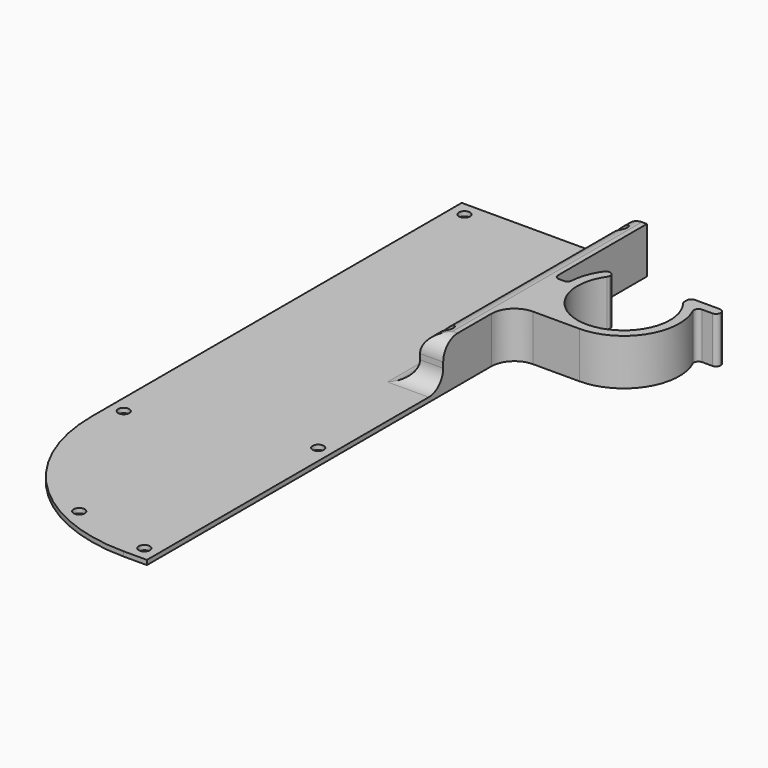
from build123d import *

# Parameters (mm, degrees)
F1_DEPTH     = 10
F3_DEPTH     = 9
F5_D         = 2.4
F6_T1_DEPTH  = 55
F6_T3_DEPTH  = 5
F6_T9_DEPTH  = 64.75
F6_T13_DEPTH = 14.75
F6_T16_DEPTH = 24.5
F6_T18_DEPTH = 74.5


# Not quite as in the source:
# - a fillet or chamfer that OpenCascade refuses, or shapes differently, is made with other operations: its cross-section is extruded or revolved along the edge and cut away or added
# - a feature names something its author has since deleted; it is built from what else it names


with BuildPart() as f1:
    # F0 (on Top) → F1 (new body)
    with BuildSketch(Plane.XY):
        with BuildLine():
            Line((-30, 0), (-70, 0))
            Line((-70, 0), (-70, -100))
            ThreePointArc((-70, -100), (-59.7487373415, -124.7487373415), (-35, -135))
            Line((-35, -135), (-30, -135))
            Line((-30, -135), (-30, -42))
            ThreePointArc((-30, -42), (-28.5355339059, -38.4644660941), (-25, -37))
            Line((-25, -37), (-15, -37))
            ThreePointArc((-15, -37), (-4.9050660078, -31.4878584828), (-4.0842494776, -20.0153846154))
            ThreePointArc((-4.0842494776, -20.0153846154), (-4.0158481001, -19.0593451264), (-3.1746036007, -18.6))
            Line((-3.1746036007, -18.6), (-1, -18.6))
            ThreePointArc((-1, -18.6), (-0.2928932188, -18.3071067812), (0, -17.6))
            ThreePointArc((0, -17.6), (-0.2928932188, -16.8928932188), (-1, -16.6))
            Line((-1, -16.6), (-6.3162509151, -16.6))
            ThreePointArc((-6.3162509151, -16.6), (-7.0233576963, -16.8928932188), (-7.3162509151, -17.6))
            Line((-7.3162509151, -17.6), (-7.3162509151, -18.2477780079))
            ThreePointArc((-7.3162509151, -18.2477780079), (-7.2621451309, -18.5722531726), (-7.1056826501, -18.8616163708))
            ThreePointArc((-7.1056826501, -18.8616163708), (-14.7582290616, -34.9970769134), (-23.1818181818, -19.2504042542))
            ThreePointArc((-23.1818181818, -19.2504042542), (-23.0465374108, -18.9769560242), (-23, -18.6754446797))
            ThreePointArc((-23, -18.6754446797), (-23.6984886554, -17.7219820904), (-24.8181818182, -18.1004851051))
            ThreePointArc((-24.8181818182, -18.1004851051), (-26.2938104102, -20.9441589751), (-26.9644443663, -24.0769230769))
            ThreePointArc((-26.9644443663, -24.0769230769), (-27.2821151763, -24.7337993857), (-27.9614813968, -25))
            Line((-27.9614813968, -25), (-29, -25))
            ThreePointArc((-29, -25), (-29.7071067812, -24.7071067812), (-30, -24))
            Line((-30, -24), (-30, 0))
        make_face()
    extrude(amount=F1_DEPTH)

    # F2 (on face) → F3 (cut)
    with BuildSketch(Plane.XY.offset(10)):
        with BuildLine():
            Line((-35, -55), (-35, 0))
            Line((-35, 0), (-70, 0))
            Line((-70, 0), (-70, -100))
            ThreePointArc((-70, -100), (-59.7487373415, -124.7487373415), (-35, -135))
            Line((-35, -135), (-30, -135))
            Line((-30, -135), (-30, -55))
            Line((-30, -55), (-35, -55))
        make_face()
    extrude(amount=-F3_DEPTH, mode=Mode.SUBTRACT)

    # F5 (through all)
    with Locations(Plane.XY.offset(10)):
        with Locations((-67, -3), (-50, -128.2665880502), (-33, -131.9374388453), (-33, -85), (-33, -50), (-33, -3), (-67, -95)):
            Hole(F5_D / 2)

    # F6: fillet of radius 3.9 on 4 edges, made by hand

    # F6_s2 → F6_t1 (join)
    with BuildSketch(Plane.XZ):
        with BuildLine():
            ThreePointArc((-35, 4.9), (-36.1422835534, 2.1422835534), (-38.9, 1))
            Line((-38.9, 1), (-35, 1))
            Line((-35, 1), (-35, 4.9))
        make_face()
    extrude(amount=F6_T1_DEPTH)

    # F6_s4 → F6_t3 (join)
    with BuildSketch(Plane.YZ.offset(-35)):
        with BuildLine():
            ThreePointArc((-55, 4.9), (-56.1422835534, 2.1422835534), (-58.9, 1))
            Line((-58.9, 1), (-55, 1))
            Line((-55, 1), (-55, 4.9))
        make_face()
    extrude(amount=F6_T3_DEPTH)


with BuildPart() as f6_tool7:
    # F6_s8 → F6_t9 (new body)
    with BuildSketch(Plane.XZ.offset(64.75)):
        with BuildLine():
            ThreePointArc((-35, 4.9), (-36.1422835534, 2.1422835534), (-38.9, 1))
            Line((-38.9, 1), (-35, 1))
            Line((-35, 1), (-35, 4.9))
        make_face()
    extrude(amount=-F6_T9_DEPTH)

    split(bisect_by=Plane.XZ.offset(55), keep=Keep.TOP)


with BuildPart() as f6_tool11:
    # F6_s12 → F6_t13 (new body)
    with BuildSketch(Plane.YZ.offset(-30)):
        with BuildLine():
            ThreePointArc((-55, 4.9), (-56.1422835534, 2.1422835534), (-58.9, 1))
            Line((-58.9, 1), (-55, 1))
            Line((-55, 1), (-55, 4.9))
        make_face()
    extrude(amount=-F6_T13_DEPTH)

    split(bisect_by=Plane.YZ.offset(-35), keep=Keep.BOTTOM)


with BuildPart() as f6_tool7_1:
    add(f6_tool7.part)

    # F6_t15: intersect F6_tool11
    add(f6_tool11.part, mode=Mode.INTERSECT)


with BuildPart() as f1_1:
    add(f1.part)

    # F6_t5: union F6_tool7
    add(f6_tool7_1.part)

    # F6_s17 → F6_t16 (cut)
    with BuildSketch(Plane.YZ.offset(-44.75)):
        with BuildLine():
            ThreePointArc((-55, 6.1), (-53.8577164466, 8.8577164466), (-51.1, 10))
            Line((-51.1, 10), (-55, 10))
            Line((-55, 10), (-55, 6.1))
        make_face()
    extrude(amount=F6_T16_DEPTH, mode=Mode.SUBTRACT)

    # F6_s19 → F6_t18 (cut)
    with BuildSketch(Plane.XZ.offset(-9.75)):
        with BuildLine():
            ThreePointArc((-35, 6.1), (-33.8577164466, 8.8577164466), (-31.1, 10))
            Line((-31.1, 10), (-35, 10))
            Line((-35, 10), (-35, 6.1))
        make_face()
    extrude(amount=F6_T18_DEPTH, mode=Mode.SUBTRACT)


solid = f1_1.part
